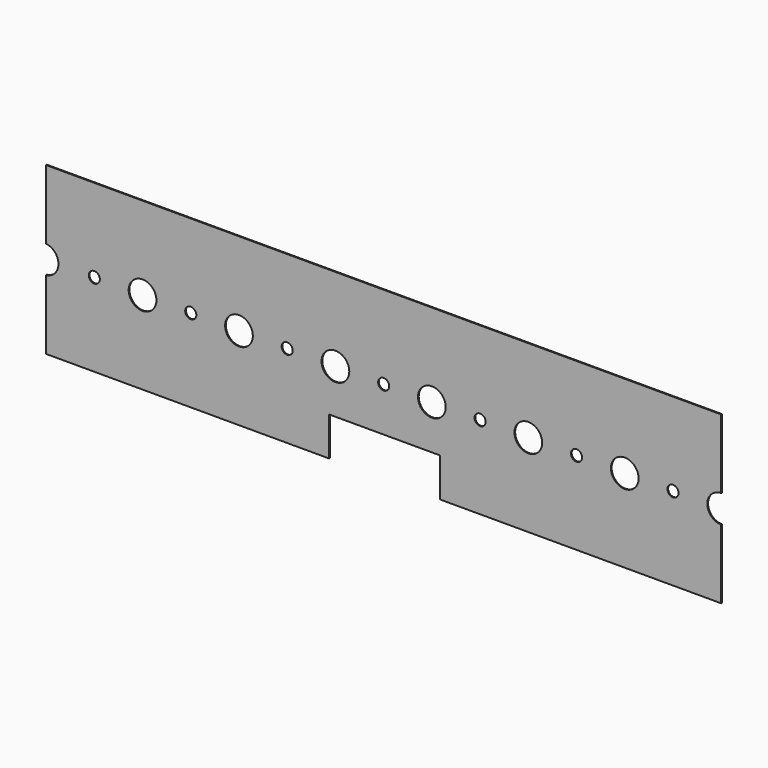
from build123d import *

# Parameters (mm, degrees)
F1_DEPTH = 0.8
F3_DEPTH = 25


# Not quite as in the source:
# - a feature names something its author has since deleted; it is built from what else it names


with BuildPart() as f1:
    # F0 (on Front) → F1 (new body, symmetric)
    with BuildSketch(Plane.XZ):
        Polygon((609, -150), (609, 150), (-609, 150), (-609, -150), (-98.2216194272, -150), (-98.2216194272, -80), (101.7783805728, -80), (101.7783805728, -150), align=None)
    extrude(amount=F1_DEPTH, both=True)

    # F2 (on face) → F3 (cut)
    with BuildSketch(Plane.XZ.offset(0.8)):
        with BuildLine():
            Line((-609, 0), (-586.7130714899, 0))
            ThreePointArc((-586.7130714899, 0), (-593.05140569, 16.7836636007), (-609, 25))
            Line((-609, 25), (-609, 0))
        make_face()
        with BuildLine():
            ThreePointArc((-460, 0), (-435, -25), (-410, 0))
            Line((-410, 0), (-435, 0))
            Line((-435, 0), (-460, 0))
        make_face()
        with BuildLine():
            Line((-435, 0), (-410, 0))
            ThreePointArc((-410, 0), (-435, 25), (-460, 0))
            Line((-460, 0), (-435, 0))
        make_face()
        with BuildLine():
            ThreePointArc((-286, 0), (-261, -25), (-236, 0))
            Line((-236, 0), (-261, 0))
            Line((-261, 0), (-286, 0))
        make_face()
        with BuildLine():
            Line((-261, 0), (-236, 0))
            ThreePointArc((-236, 0), (-261, 25), (-286, 0))
            Line((-286, 0), (-261, 0))
        make_face()
        with BuildLine():
            ThreePointArc((-112, 0), (-87, -25), (-62, 0))
            Line((-62, 0), (-87, 0))
            Line((-87, 0), (-112, 0))
        make_face()
        with BuildLine():
            Line((-87, 0), (-62, 0))
            ThreePointArc((-62, 0), (-87, 25), (-112, 0))
            Line((-112, 0), (-87, 0))
        make_face()
        with BuildLine():
            ThreePointArc((112, 0), (87, 25), (62, 0))
            Line((62, 0), (87, 0))
            Line((87, 0), (112, 0))
        make_face()
        with BuildLine():
            Line((87, 0), (62, 0))
            ThreePointArc((62, 0), (87, -25), (112, 0))
            Line((112, 0), (87, 0))
        make_face()
        with BuildLine():
            ThreePointArc((286, 0), (261, 25), (236, 0))
            Line((236, 0), (261, 0))
            Line((261, 0), (286, 0))
        make_face()
        with BuildLine():
            Line((261, 0), (236, 0))
            ThreePointArc((236, 0), (261, -25), (286, 0))
            Line((286, 0), (261, 0))
        make_face()
        with BuildLine():
            ThreePointArc((460, 0), (435, 25), (410, 0))
            Line((410, 0), (435, 0))
            Line((435, 0), (460, 0))
        make_face()
        with BuildLine():
            Line((435, 0), (410, 0))
            ThreePointArc((410, 0), (435, -25), (460, 0))
            Line((460, 0), (435, 0))
        make_face()
        with BuildLine():
            ThreePointArc((-609, -24.7047928188), (-593.1499526355, -16.5983450419), (-586.7130714899, 0))
            Line((-586.7130714899, 0), (-609, 0))
            Line((-609, 0), (-609, -24.7047928188))
        make_face()
        with BuildLine():
            ThreePointArc((609, 25), (591.3223304703, 17.6776695297), (584, 0))
            Line((584, 0), (609, 0))
            Line((609, 0), (609, 25))
        make_face()
        with BuildLine():
            Line((609, 0), (584, 0))
            ThreePointArc((584, 0), (591.3223304703, -17.6776695297), (609, -25))
            Line((609, -25), (609, 0))
        make_face()
        with BuildLine():
            ThreePointArc((-532, 0), (-522, -10), (-512, 0))
            Line((-512, 0), (-532, 0))
        make_face()
        with BuildLine():
            Line((-532, 0), (-512, 0))
            ThreePointArc((-512, 0), (-522, 10), (-532, 0))
        make_face()
        with BuildLine():
            ThreePointArc((-358, 0), (-348, -10), (-338, 0))
            Line((-338, 0), (-358, 0))
        make_face()
        with BuildLine():
            Line((-358, 0), (-338, 0))
            ThreePointArc((-338, 0), (-348, 10), (-358, 0))
        make_face()
        with BuildLine():
            ThreePointArc((-184, 0), (-174, -10), (-164, 0))
            Line((-164, 0), (-184, 0))
        make_face()
        with BuildLine():
            Line((-184, 0), (-164, 0))
            ThreePointArc((-164, 0), (-174, 10), (-184, 0))
        make_face()
        with BuildLine():
            Line((0, 0), (-10, 0))
            ThreePointArc((-10, 0), (0, -10), (10, 0))
            Line((10, 0), (0, 0))
        make_face()
        with BuildLine():
            ThreePointArc((10, 0), (0, 10), (-10, 0))
            Line((-10, 0), (0, 0))
            Line((0, 0), (10, 0))
        make_face()
        with BuildLine():
            ThreePointArc((184, 0), (174, 10), (164, 0))
            Line((164, 0), (184, 0))
        make_face()
        with BuildLine():
            Line((184, 0), (164, 0))
            ThreePointArc((164, 0), (174, -10), (184, 0))
        make_face()
        with BuildLine():
            ThreePointArc((358, 0), (348, 10), (338, 0))
            Line((338, 0), (358, 0))
        make_face()
        with BuildLine():
            Line((358, 0), (338, 0))
            ThreePointArc((338, 0), (348, -10), (358, 0))
        make_face()
        with BuildLine():
            ThreePointArc((532, 0), (522, 10), (512, 0))
            Line((512, 0), (532, 0))
        make_face()
        with BuildLine():
            Line((532, 0), (512, 0))
            ThreePointArc((512, 0), (522, -10), (532, 0))
        make_face()
    extrude(amount=-F3_DEPTH, mode=Mode.SUBTRACT)


solid = f1.part
